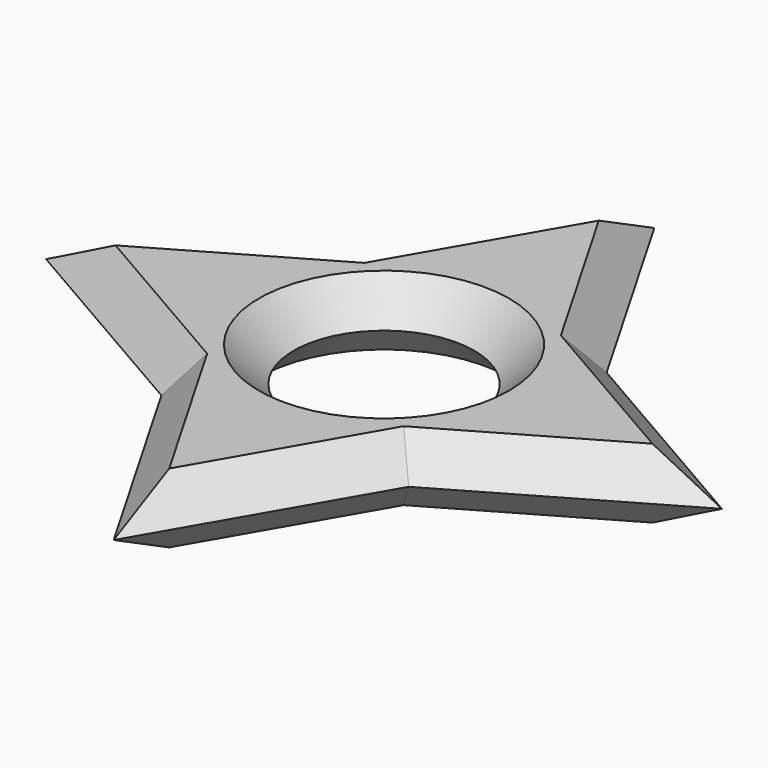
from build123d import *

# Parameters (mm, degrees)
F0_W         = 25.4
F0_H         = 25.4
F0_R         = 6.35
F1_DEPTH     = 6.35
F2_SIZE      = 5.08
F3_T4_DEPTH  = 51.5282991577
F3_T9_DEPTH  = 51.5282991577
F3_T14_DEPTH = 51.5282991577
F3_T19_DEPTH = 51.5282991577
F3_T24_DEPTH = 51.5282991577
F3_T29_DEPTH = 51.5282991577
F3_T34_DEPTH = 51.5282991577
F3_T39_DEPTH = 51.5282991577
F3_T47_DEPTH = 51.5282991577
F3_T51_DEPTH = 51.5282991577
F3_T58_DEPTH = 51.5282991577
F3_T62_DEPTH = 51.5282991577
F3_T69_DEPTH = 51.5282991577
F3_T73_DEPTH = 51.5282991577
F3_T80_DEPTH = 51.5282991577
F3_T84_DEPTH = 51.5282991577


# Not quite as in the source:
# - a fillet or chamfer that OpenCascade refuses, or shapes differently, is made with other operations: its cross-section is extruded or revolved along the edge and cut away or added


with BuildPart() as f1:
    # F0 (on Top) → F1 (new body)
    with BuildSketch(Plane.XY):
        Polygon((12.7, 47.3970452561), (0, 25.4), (25.4, 25.4), align=None)
        with Locations((12.7, 12.7)):
            Rectangle(F0_W, F0_H)
        with Locations((12.7, 12.7)):
            Circle(F0_R, mode=Mode.SUBTRACT)
        Polygon((25.4, 25.4), (25.4, 0), (47.3970452561, 12.7), align=None)
        Polygon((25.4, 0), (0, 0), (12.7, -21.9970452561), align=None)
        Polygon((-21.9970452561, 12.7), (0, 0), (0, 25.4), align=None)
    extrude(amount=F1_DEPTH)

    # F2
    f2_edges = [f1.edges().sort_by_distance(p)[0] for p in [
        (6.35, 36.398523, 6.35),
        (-10.998523, 19.05, 6.35),
        (-10.998523, 6.35, 6.35),
        (6.35, -10.998523, 6.35),
        (19.05, -10.998523, 6.35),
        (36.398523, 6.35, 6.35),
        (36.398523, 19.05, 6.35),
        (19.05, 36.398523, 6.35),
        (6.35, 12.7, 6.35),
    ]]
    chamfer(f2_edges, length=F2_SIZE)

    # F3: chamfer of 5.08 on 9 edges, made by hand


with BuildPart() as f3_tool2:
    # F3_s3 → F3_t4 (new body)
    with BuildSketch(Plane(origin=(41.3624080422, -23.8805974175, 0), x_dir=(0, 0, 1), z_dir=(-0.8660254038, 0.5, 0))):
        Polygon((0, 29.6170452561), (5.08, 34.6970452561), (0, 34.6970452561), align=None)
    extrude(amount=F3_T4_DEPTH)

    split(bisect_by=Plane(origin=(30.0485226281, 17.3485226281, 0), x_dir=(0, 0, 1), z_dir=(0.8660254038, 0.5, 0)), keep=Keep.TOP)


with BuildPart() as f1_1:
    add(f1.part)

    # F3_t1: cut F3_tool2
    add(f3_tool2.part, mode=Mode.SUBTRACT)


with BuildPart() as f3_tool7:
    # F3_s8 → F3_t9 (new body)
    with BuildSketch(Plane(origin=(30.2305974175, 52.3609306703, 0), x_dir=(0, 0, 1), z_dir=(-0.5, -0.8660254038, 0))):
        Polygon((5.08, 12.7), (0, 7.62), (0, 12.7), align=None)
    extrude(amount=F3_T9_DEPTH)

    split(bisect_by=Plane(origin=(-10.9985226281, 19.05, 0), x_dir=(0, 0, 1), z_dir=(-0.5, 0.8660254038, 0)), keep=Keep.TOP)


with BuildPart() as f1_2:
    add(f1_1.part)

    # F3_t6: cut F3_tool7
    add(f3_tool7.part, mode=Mode.SUBTRACT)


with BuildPart() as f3_tool12:
    # F3_s13 → F3_t14 (new body)
    with BuildSketch(Plane(origin=(22.3124080422, 12.8820747894, 0), x_dir=(0, 0, 1), z_dir=(-0.8660254038, -0.5, 0))):
        Polygon((0, 16.9170452561), (5.08, 21.9970452561), (0, 21.9970452561), align=None)
    extrude(amount=F3_T14_DEPTH)

    split(bisect_by=Plane(origin=(-10.9985226281, 6.35, 0), x_dir=(0, 0, 1), z_dir=(-0.8660254038, 0.5, 0)), keep=Keep.TOP)


with BuildPart() as f1_3:
    add(f1_2.part)

    # F3_t11: cut F3_tool12
    add(f3_tool12.part, mode=Mode.SUBTRACT)


with BuildPart() as f3_tool17:
    # F3_s18 → F3_t19 (new body)
    with BuildSketch(Plane(origin=(-33.3109306703, 19.2320747894, 0), x_dir=(0, 0, 1), z_dir=(0.8660254038, -0.5, 0))):
        Polygon((0, -5.08), (5.08, 0), (0, 0), align=None)
    extrude(amount=F3_T19_DEPTH)

    split(bisect_by=Plane(origin=(0, 0, 0), x_dir=(0, 0, 1), z_dir=(-0.8660254038, -0.5, 0)), keep=Keep.TOP)


with BuildPart() as f1_4:
    add(f1_3.part)

    # F3_t16: cut F3_tool17
    add(f3_tool17.part, mode=Mode.SUBTRACT)


with BuildPart() as f3_tool22:
    # F3_s23 → F3_t24 (new body)
    with BuildSketch(Plane(origin=(-6.5320747894, 11.3138854141, 0), x_dir=(0, 0, 1), z_dir=(0.5, -0.8660254038, 0))):
        Polygon((0, -5.08), (5.08, 0), (0, 0), align=None)
    extrude(amount=F3_T24_DEPTH)

    split(bisect_by=Plane(origin=(0, 0, 0), x_dir=(0, 0, 1), z_dir=(-0.5, -0.8660254038, 0)), keep=Keep.TOP)


with BuildPart() as f1_5:
    add(f1_4.part)

    # F3_t21: cut F3_tool22
    add(f3_tool22.part, mode=Mode.SUBTRACT)


with BuildPart() as f3_tool27:
    # F3_s28 → F3_t29 (new body)
    with BuildSketch(Plane(origin=(-12.8820747894, -22.3124080422, 0), x_dir=(0, 0, 1), z_dir=(0.5, 0.8660254038, 0))):
        Polygon((0, 16.9170452561), (5.08, 21.9970452561), (0, 21.9970452561), align=None)
    extrude(amount=F3_T29_DEPTH)

    split(bisect_by=Plane(origin=(6.35, -10.9985226281, 0), x_dir=(0, 0, 1), z_dir=(0.5, -0.8660254038, 0)), keep=Keep.TOP)


with BuildPart() as f1_6:
    add(f1_5.part)

    # F3_t26: cut F3_tool27
    add(f3_tool27.part, mode=Mode.SUBTRACT)


with BuildPart() as f3_tool32:
    # F3_s33 → F3_t34 (new body)
    with BuildSketch(Plane(origin=(7.7361145859, 4.4664478386, 0), x_dir=(0, 0, 1), z_dir=(0.8660254038, 0.5, 0))):
        Polygon((0, 7.62), (5.08, 12.7), (0, 12.7), align=None)
    extrude(amount=F3_T34_DEPTH)

    split(bisect_by=Plane(origin=(19.05, -10.9985226281, 0), x_dir=(0, 0, 1), z_dir=(0.8660254038, -0.5, 0)), keep=Keep.TOP)


with BuildPart() as f1_7:
    add(f1_6.part)

    # F3_t31: cut F3_tool32
    add(f3_tool32.part, mode=Mode.SUBTRACT)


with BuildPart() as f3_tool37:
    # F3_s38 → F3_t39 (new body)
    with BuildSketch(Plane(origin=(1.8835521614, -3.2624080422, 0), x_dir=(0, 0, 1), z_dir=(-0.5, 0.8660254038, 0))):
        Polygon((5.08, 34.6970452561), (0, 29.6170452561), (0, 34.6970452561), align=None)
    extrude(amount=F3_T39_DEPTH)

    split(bisect_by=Plane(origin=(17.3485226281, 30.0485226281, 0), x_dir=(0, 0, 1), z_dir=(0.5, 0.8660254038, 0)), keep=Keep.TOP)


with BuildPart() as f1_8:
    add(f1_7.part)

    # F3_t36: cut F3_tool37
    add(f3_tool37.part, mode=Mode.SUBTRACT)

    # F3_s41 → F3_t42 (revolve, cut)
    with BuildSketch(Plane.XZ.offset(-12.7)):
        Polygon((24.13, 0), (19.05, 5.08), (19.05, 0), align=None)
    revolve(axis=Axis((12.7, 12.7, 0), (0, 0, 1)), mode=Mode.SUBTRACT)


with BuildPart() as f3_tool45:
    # F3_s46 → F3_t47 (new body)
    with BuildSketch(Plane(origin=(1.8835521614, -3.2624080422, 0), x_dir=(0, 0, 1), z_dir=(-0.5, 0.8660254038, 0))):
        Polygon((5.08, 34.6970452561), (0, 29.6170452561), (0, 34.6970452561), align=None)
    extrude(amount=F3_T47_DEPTH)

    split(bisect_by=Plane(origin=(17.3485226281, 30.0485226281, 0), x_dir=(0, 0, 1), z_dir=(-0.5, -0.8660254038, 0)), keep=Keep.TOP)


with BuildPart() as f3_tool49:
    # F3_s50 → F3_t51 (new body)
    with BuildSketch(Plane(origin=(41.3624080422, -23.8805974175, 0), x_dir=(0, 0, 1), z_dir=(-0.8660254038, 0.5, 0))):
        Polygon((0, 29.6170452561), (5.08, 34.6970452561), (0, 34.6970452561), align=None)
    extrude(amount=F3_T51_DEPTH)

    split(bisect_by=Plane(origin=(30.0485226281, 17.3485226281, 0), x_dir=(0, 0, 1), z_dir=(-0.8660254038, -0.5, 0)), keep=Keep.TOP)


with BuildPart() as f3_tool45_1:
    add(f3_tool45.part)

    # F3_t53: intersect F3_tool49
    add(f3_tool49.part, mode=Mode.INTERSECT)


with BuildPart() as f1_9:
    add(f1_8.part)

    # F3_t43: cut F3_tool45
    add(f3_tool45_1.part, mode=Mode.SUBTRACT)


with BuildPart() as f3_tool56:
    # F3_s57 → F3_t58 (new body)
    with BuildSketch(Plane(origin=(30.2305974175, 52.3609306703, 0), x_dir=(0, 0, 1), z_dir=(-0.5, -0.8660254038, 0))):
        Polygon((5.08, 12.7), (0, 7.62), (0, 12.7), align=None)
    extrude(amount=F3_T58_DEPTH)

    split(bisect_by=Plane(origin=(-10.9985226281, 19.05, 0), x_dir=(0, 0, 1), z_dir=(0.5, -0.8660254038, 0)), keep=Keep.TOP)


with BuildPart() as f3_tool60:
    # F3_s61 → F3_t62 (new body)
    with BuildSketch(Plane(origin=(22.3124080422, 12.8820747894, 0), x_dir=(0, 0, 1), z_dir=(-0.8660254038, -0.5, 0))):
        Polygon((0, 16.9170452561), (5.08, 21.9970452561), (0, 21.9970452561), align=None)
    extrude(amount=F3_T62_DEPTH)

    split(bisect_by=Plane(origin=(-10.9985226281, 6.35, 0), x_dir=(0, 0, 1), z_dir=(0.8660254038, -0.5, 0)), keep=Keep.TOP)


with BuildPart() as f3_tool56_1:
    add(f3_tool56.part)

    # F3_t64: intersect F3_tool60
    add(f3_tool60.part, mode=Mode.INTERSECT)


with BuildPart() as f1_10:
    add(f1_9.part)

    # F3_t54: cut F3_tool56
    add(f3_tool56_1.part, mode=Mode.SUBTRACT)


with BuildPart() as f3_tool67:
    # F3_s68 → F3_t69 (new body)
    with BuildSketch(Plane(origin=(-33.3109306703, 19.2320747894, 0), x_dir=(0, 0, 1), z_dir=(0.8660254038, -0.5, 0))):
        Polygon((0, -5.08), (5.08, 0), (0, 0), align=None)
    extrude(amount=F3_T69_DEPTH)

    split(bisect_by=Plane(origin=(0, 0, 0), x_dir=(0, 0, 1), z_dir=(0.8660254038, 0.5, 0)), keep=Keep.TOP)


with BuildPart() as f3_tool71:
    # F3_s72 → F3_t73 (new body)
    with BuildSketch(Plane(origin=(-6.5320747894, 11.3138854141, 0), x_dir=(0, 0, 1), z_dir=(0.5, -0.8660254038, 0))):
        Polygon((0, -5.08), (5.08, 0), (0, 0), align=None)
    extrude(amount=F3_T73_DEPTH)

    split(bisect_by=Plane(origin=(0, 0, 0), x_dir=(0, 0, 1), z_dir=(0.5, 0.8660254038, 0)), keep=Keep.TOP)


with BuildPart() as f3_tool67_1:
    add(f3_tool67.part)

    # F3_t75: intersect F3_tool71
    add(f3_tool71.part, mode=Mode.INTERSECT)


with BuildPart() as f1_11:
    add(f1_10.part)

    # F3_t65: cut F3_tool67
    add(f3_tool67_1.part, mode=Mode.SUBTRACT)


with BuildPart() as f3_tool78:
    # F3_s79 → F3_t80 (new body)
    with BuildSketch(Plane(origin=(-12.8820747894, -22.3124080422, 0), x_dir=(0, 0, 1), z_dir=(0.5, 0.8660254038, 0))):
        Polygon((0, 16.9170452561), (5.08, 21.9970452561), (0, 21.9970452561), align=None)
    extrude(amount=F3_T80_DEPTH)

    split(bisect_by=Plane(origin=(6.35, -10.9985226281, 0), x_dir=(0, 0, 1), z_dir=(-0.5, 0.8660254038, 0)), keep=Keep.TOP)


with BuildPart() as f3_tool82:
    # F3_s83 → F3_t84 (new body)
    with BuildSketch(Plane(origin=(7.7361145859, 4.4664478386, 0), x_dir=(0, 0, 1), z_dir=(0.8660254038, 0.5, 0))):
        Polygon((0, 7.62), (5.08, 12.7), (0, 12.7), align=None)
    extrude(amount=F3_T84_DEPTH)

    split(bisect_by=Plane(origin=(19.05, -10.9985226281, 0), x_dir=(0, 0, 1), z_dir=(-0.8660254038, 0.5, 0)), keep=Keep.TOP)


with BuildPart() as f3_tool78_1:
    add(f3_tool78.part)

    # F3_t86: intersect F3_tool82
    add(f3_tool82.part, mode=Mode.INTERSECT)


with BuildPart() as f1_12:
    add(f1_11.part)

    # F3_t76: cut F3_tool78
    add(f3_tool78_1.part, mode=Mode.SUBTRACT)


solid = f1_12.part
